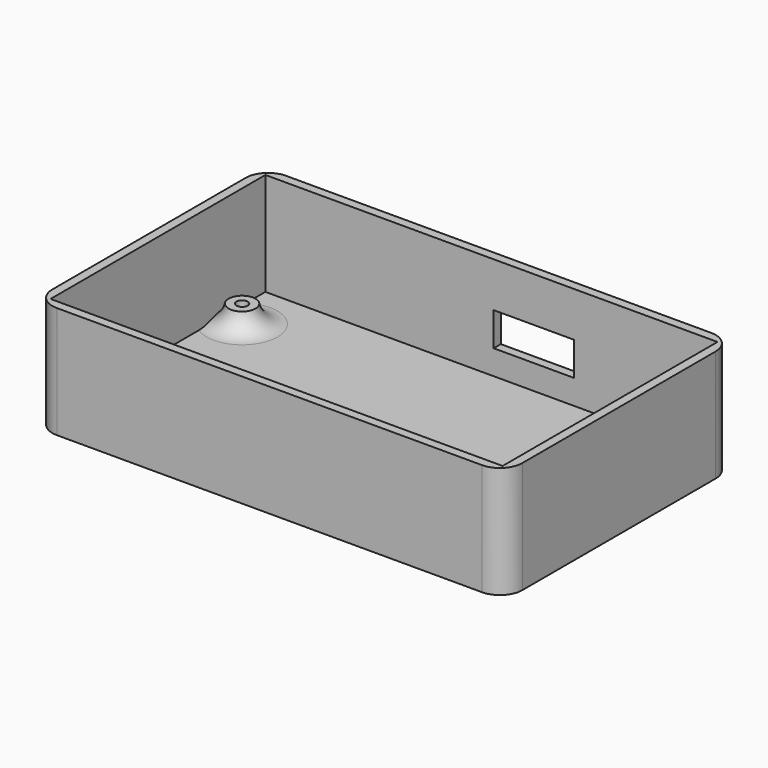
from build123d import *

# Parameters (mm, degrees)
F0_W         = 101
F0_H         = 60
F1_DEPTH     = 2
F2_W         = 105
F2_H         = 64
F2_W_2       = 101
F2_H_2       = 60
F3_DEPTH     = 25
F4_R         = 3
F4_R_2       = 1.25
F5_DEPTH     = 6
F6_W         = 18
F6_H         = 7.5
F7_DEPTH     = 5
F8_T15_DEPTH = 50


# Not quite as in the source:
# - a fillet or chamfer that OpenCascade refuses, or shapes differently, is made with other operations: its cross-section is extruded or revolved along the edge and cut away or added


with BuildPart() as f1:
    # F0 (on Top) → F1 (new body)
    with BuildSketch(Plane.XY):
        Rectangle(F0_W, F0_H)
    extrude(amount=F1_DEPTH)

    # F2 (on Top) → F3 (join)
    with BuildSketch(Plane.XY):
        Rectangle(F2_W, F2_H)
        Rectangle(F2_W_2, F2_H_2, mode=Mode.SUBTRACT)
    extrude(amount=F3_DEPTH)

    # F4 (on Top) → F5 (join)
    with BuildSketch(Plane.XY):
        with Locations((-46.1, 18)):
            Circle(F4_R)
        with Locations((-46.1, 18)):
            Circle(F4_R_2, mode=Mode.SUBTRACT)
        with Locations((-46.1, -21)):
            Circle(F4_R)
        with Locations((-46.1, -21)):
            Circle(F4_R_2, mode=Mode.SUBTRACT)
        with Locations((43.5, -21)):
            Circle(F4_R)
        with Locations((43.5, -21)):
            Circle(F4_R_2, mode=Mode.SUBTRACT)
        with Locations((43.5, 18)):
            Circle(F4_R)
        with Locations((43.5, 18)):
            Circle(F4_R_2, mode=Mode.SUBTRACT)
    extrude(amount=F5_DEPTH)

    # F6 (on face) → F7 (cut)
    with BuildSketch(Plane(origin=(0, 32, 0), x_dir=(-1, 0, 0), z_dir=(0, 1, 0))):
        with Locations((-9.5, 11.25)):
            Rectangle(F6_W, F6_H)
    extrude(amount=-F7_DEPTH, mode=Mode.SUBTRACT)

    # F8: fillet of radius 5 on 8 edges, made by hand

    # F8_s1 → F8_t2 (revolve)
    with BuildSketch(Plane.XZ.offset(21)):
        with BuildLine():
            ThreePointArc((51.3989794856, 2), (48.2367018254, 3.1270166538), (46.5, 6))
            Line((46.5, 6), (46.5, 2))
            Line((46.5, 2), (51.3989794856, 2))
        make_face()
    revolve(axis=Axis((43.5, -21, 2), (0, 0, -1)))

    # F8_s3 → F8_t4 (revolve)
    with BuildSketch(Plane.XZ.offset(-18)):
        with BuildLine():
            ThreePointArc((51.3989794856, 2), (48.2367018254, 3.1270166538), (46.5, 6))
            Line((46.5, 6), (46.5, 2))
            Line((46.5, 2), (51.3989794856, 2))
        make_face()
    revolve(axis=Axis((43.5, 18, 2), (0, 0, -1)))


with BuildPart() as f8_tool6:
    # F8_s7 → F8_t8 (revolve)
    with BuildSketch(Plane.XZ.offset(21)):
        with BuildLine():
            ThreePointArc((-38.2010205144, 2), (-41.3632981746, 3.1270166538), (-43.1, 6))
            Line((-43.1, 6), (-43.1, 2))
            Line((-43.1, 2), (-38.2010205144, 2))
        make_face()
    revolve(axis=Axis((-46.1, -21, 2), (0, 0, -1)))

    split(bisect_by=Plane.YZ.offset(-50.5), keep=Keep.TOP)


with BuildPart() as f1_1:
    add(f1.part)

    # F8_t5: union F8_tool6
    add(f8_tool6.part)


with BuildPart() as f8_tool11:
    # F8_s12 → F8_t13 (revolve)
    with BuildSketch(Plane.XZ.offset(-18)):
        with BuildLine():
            ThreePointArc((-38.2010205144, 2), (-41.3632981746, 3.1270166538), (-43.1, 6))
            Line((-43.1, 6), (-43.1, 2))
            Line((-43.1, 2), (-38.2010205144, 2))
        make_face()
    revolve(axis=Axis((-46.1, 18, 2), (0, 0, -1)))

    split(bisect_by=Plane.YZ.offset(-50.5), keep=Keep.TOP)


with BuildPart() as f1_2:
    add(f1_1.part)

    # F8_t10: union F8_tool11
    add(f8_tool11.part)

    # F8_s16 → F8_t15 (cut)
    with BuildSketch(Plane.XY.offset(-12.5)):
        with BuildLine():
            ThreePointArc((-47.5, 32), (-51.0355339059, 30.5355339059), (-52.5, 27))
            Line((-52.5, 27), (-52.5, 32))
            Line((-52.5, 32), (-47.5, 32))
        make_face()
        with BuildLine():
            ThreePointArc((-47.5, -32), (-51.0355339059, -30.5355339059), (-52.5, -27))
            Line((-52.5, -27), (-52.5, -32))
            Line((-52.5, -32), (-47.5, -32))
        make_face()
        with BuildLine():
            ThreePointArc((47.5, -32), (51.0355339059, -30.5355339059), (52.5, -27))
            Line((52.5, -27), (52.5, -32))
            Line((52.5, -32), (47.5, -32))
        make_face()
        with BuildLine():
            ThreePointArc((52.5, 27), (51.0355339059, 30.5355339059), (47.5, 32))
            Line((47.5, 32), (52.5, 32))
            Line((52.5, 32), (52.5, 27))
        make_face()
    extrude(amount=F8_T15_DEPTH, mode=Mode.SUBTRACT)


solid = f1_2.part
